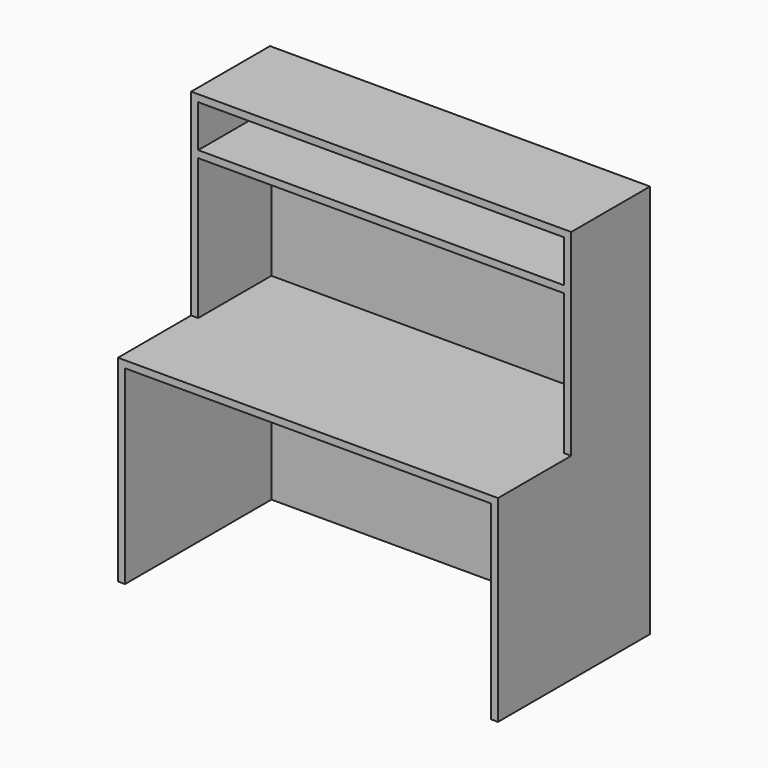
from build123d import *

# Parameters (mm, degrees)
F2_DEPTH = 6.35
F3_W     = 165.1
F3_H     = 6.35
F4_DEPTH = 165.1
F5_W     = 165.1
F5_H     = 6.35
F6_DEPTH = 82.55
F8_W     = 342.9
F8_H     = 355.6
F9_DEPTH = 6.35


with BuildPart() as f2:
    # F1 (on offset) → F2 (new body)
    with BuildSketch(Plane.YZ.offset(165.1)):
        Polygon((-82.55, 177.8), (-82.55, 0), (82.55, 0), (82.55, 355.6), (0, 355.6), (0, 177.8), align=None)
    extrude(amount=F2_DEPTH)

    # F3 (on face) → F4 (join, through all)
    with BuildSketch(Plane.XZ.offset(82.55)):
        with Locations((82.55, 174.625)):
            Rectangle(F3_W, F3_H)
    extrude(amount=-F4_DEPTH)

    # F5 (on face) → F6 (join, through all)
    with BuildSketch(Plane.XZ):
        with Locations((82.55, 352.425)):
            Rectangle(F5_W, F5_H)
        with Locations((82.55, 307.975)):
            Rectangle(F5_W, F5_H)
    extrude(amount=-F6_DEPTH)

    # F7: F2 across plane


with BuildPart() as f2_1:
    add(f2.part)
    add(f2.part.mirror(Plane.YZ))

    # F8 (on face) → F9 (join)
    with BuildSketch(Plane(origin=(0, 82.55, 0), x_dir=(-1, 0, 0), z_dir=(0, 1, 0))):
        with Locations((0, 177.8)):
            Rectangle(F8_W, F8_H)
    extrude(amount=F9_DEPTH)


solid = f2_1.part
